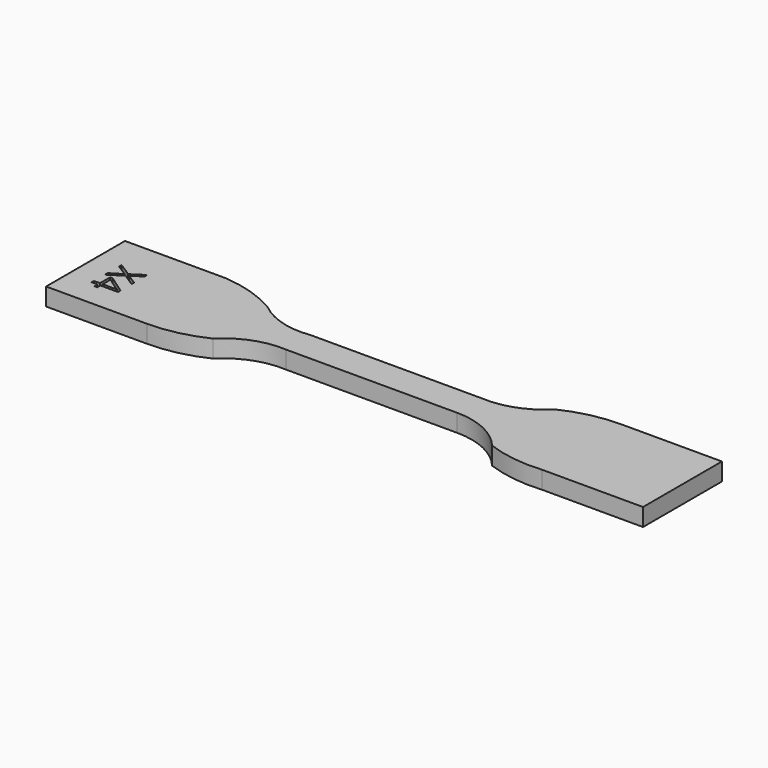
from build123d import *

# Parameters (mm, degrees)
F1_DEPTH     = 3.4
F2_TEXT_SIZE = 7.0564552314
F3_DEPTH     = 1


# Not quite as in the source:
# - Text() gives the source's letters only with a copy of the font that has no kerning and outlines rounded to 1/6400 em; it was checked with that copy


with BuildPart() as f1:
    # F0 (on Top) → F1 (new body)
    with BuildSketch(Plane.XY):
        with BuildLine():
            Line((-14.4320548165, 19.7811394548), (-33.8720548165, 19.7811394548))
            Line((-33.8720548165, 19.7811394548), (-33.8720548165, 0.7811394548))
            Line((-33.8720548165, 0.7811394548), (-14.4320548165, 0.7811394548))
            ThreePointArc((-14.4320548165, 0.7811394548), (-8.9053122052, 1.3996892086), (-3.6520548165, 3.2247301661))
            ThreePointArc((-3.6520548165, 3.2247301661), (1.3014698263, 6.4128780055), (7.1279451835, 7.2811394548))
            Line((7.1279451835, 7.2811394548), (40.1279451835, 7.2811394548))
            ThreePointArc((40.1279451835, 7.2811394548), (46.0837574042, 5.9511158081), (50.9079451835, 2.2137538538))
            ThreePointArc((50.9079451835, 2.2137538538), (56.2191047011, 0.9041953221), (61.6879451835, 0.7811394548))
            Line((61.6879451835, 0.7811394548), (81.1279451835, 0.7811394548))
            Line((81.1279451835, 0.7811394548), (81.1279451835, 19.7811394548))
            Line((81.1279451835, 19.7811394548), (61.6879451835, 19.7811394548))
            ThreePointArc((61.6879451835, 19.7811394548), (56.1612025723, 19.162589701), (50.9079451835, 17.3375487435))
            ThreePointArc((50.9079451835, 17.3375487435), (45.9544205407, 14.1494009041), (40.1279451835, 13.2811394548))
            Line((40.1279451835, 13.2811394548), (7.1279451835, 13.2811394548))
            ThreePointArc((7.1279451835, 13.2811394548), (1.4167452884, 13.6925537245), (-3.6520548165, 16.3560723447))
            ThreePointArc((-3.6520548165, 16.3560723447), (-8.8458057958, 18.686276846), (-14.4320548165, 19.7811394548))
        make_face()
    extrude(amount=F1_DEPTH)

    # F2 (on face) → F3 (cut)
    with BuildSketch(Plane.XY.offset(3.4)):
        with Locations(Location((-29.3720550835, 13.353464842), (0, 0, -90))):
            Text('X4', F2_TEXT_SIZE, font='Open Sans', text_align=(TextAlign.LEFT, TextAlign.BOTTOM))
    extrude(amount=-F3_DEPTH, mode=Mode.SUBTRACT)


solid = f1.part
